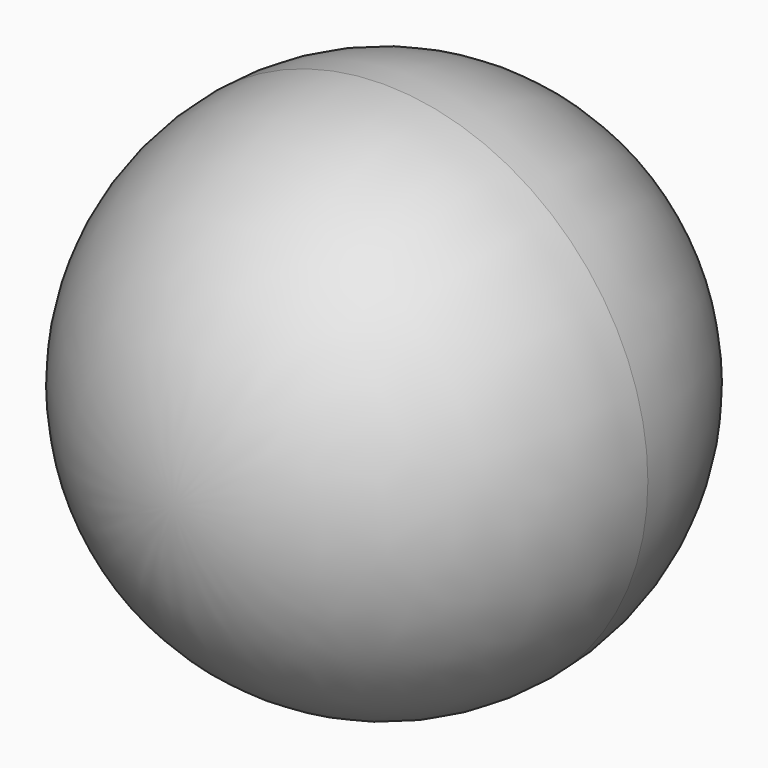
from build123d import *

# Parameters (mm, degrees)
F0_R     = 63.5
F1_DEPTH = 63.5
F2_R     = 63.49999


# Not quite as in the source:
# - a fillet or chamfer is up to 0.001 mm smaller than in the source, because OpenCascade refuses the exact size


with BuildPart() as f1:
    # F0 (on Front) → F1 (new body, symmetric)
    with BuildSketch(Plane.XZ):
        Circle(F0_R)
    extrude(amount=F1_DEPTH, both=True)

    # F2 (radius 63.5 in the source; OpenCascade refuses exactly that, so slightly less here)
    f2_edges = [f1.edges().sort_by_distance(p)[0] for p in [
        (-63.5, 63.5, 0),
        (63.5, 0, 0),
        (-63.5, -63.5, 0),
    ]]
    fillet(f2_edges, radius=F2_R)


solid = f1.part
